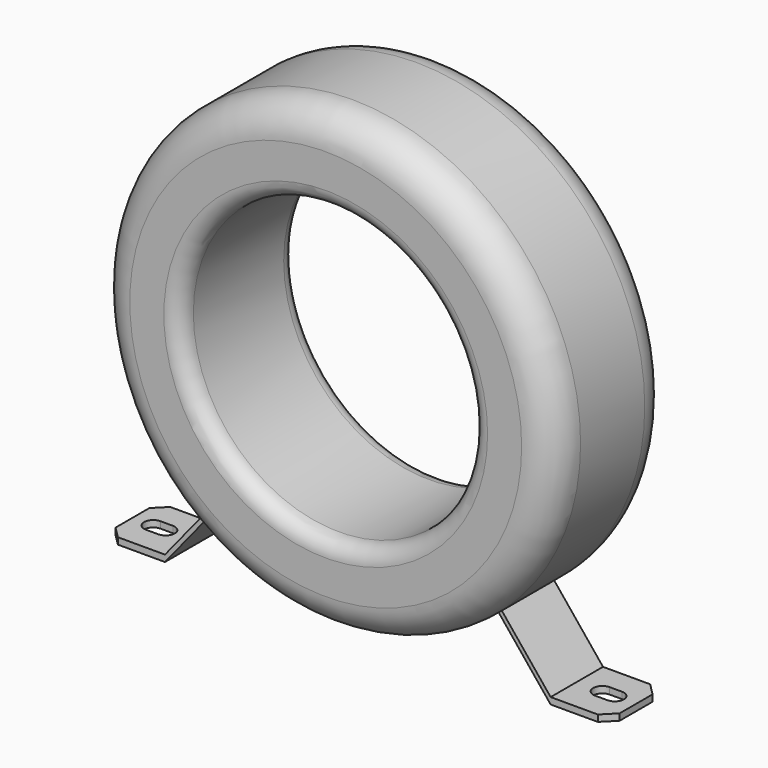
from build123d import *

# Parameters (mm, degrees)
F0_R     = 69.85
F0_R_2   = 44.45
F1_DEPTH = 22.25
F2_R     = 10
F3_R     = 5
F7_DEPTH = 2
F9_DEPTH = 20


with BuildPart() as f1:
    # F0 (on Front) → F1 (new body, symmetric)
    with BuildSketch(Plane.XZ):
        with Locations((0, 69.85)):
            Circle(F0_R)
        with Locations((0, 69.85)):
            Circle(F0_R_2, mode=Mode.SUBTRACT)
    extrude(amount=F1_DEPTH, both=True)

    # F2
    f2_edges = [f1.edges().sort_by_distance(p)[0] for p in [
        (-69.85, -22.25, 69.85),
        (-69.85, 22.25, 69.85),
    ]]
    fillet(f2_edges, radius=F2_R)

    # F3
    f3_edges = [f1.edges().sort_by_distance(p)[0] for p in [
        (-44.45, 22.25, 69.85),
        (-44.45, -22.25, 69.85),
    ]]
    fillet(f3_edges, radius=F3_R)



with BuildPart() as f7:
    # F5 (on face) → F7 (new body)
    with BuildSketch(Plane(origin=(0, 0, -4.8), x_dir=(1, 0, 0), z_dir=(0, 0, -1))):
        with BuildLine():
            Line((58.9, 10), (58.9, -10))
            Line((58.9, -10), (67.5496086478, -10))
            Line((67.5496086478, -10), (67.5496086478, -2.8))
            Line((67.5496086478, -2.8), (66.7, -2.8))
            ThreePointArc((66.7, -2.8), (63.9, 0), (66.7, 2.8))
            Line((66.7, 2.8), (67.5496086478, 2.8))
            Line((67.5496086478, 2.8), (67.5496086478, 10))
            Line((67.5496086478, 10), (58.9, 10))
        make_face()
        with BuildLine():
            Line((67.5496086478, -2.8), (67.5496086478, -10))
            Line((67.5496086478, -10), (73.3, -10))
            Line((73.3, -10), (77, -6.3))
            Line((77, -6.3), (77, 6.3))
            Line((77, 6.3), (73.3, 10))
            Line((73.3, 10), (67.5496086478, 10))
            Line((67.5496086478, 10), (67.5496086478, 2.8))
            Line((67.5496086478, 2.8), (70.5, 2.8))
            ThreePointArc((70.5, 2.8), (72.4798989873, 1.9798989873), (73.3, 0))
            ThreePointArc((73.3, 0), (72.4798989873, -1.9798989873), (70.5, -2.8))
            Line((70.5, -2.8), (67.5496086478, -2.8))
        make_face()
    extrude(amount=-F7_DEPTH)


with BuildPart() as f7b:
    # F5 (on face) → F7, piece 2 (new body)
    with BuildSketch(Plane(origin=(0, 0, -4.8), x_dir=(1, 0, 0), z_dir=(0, 0, -1))):
        Polygon((-76.8326967955, 6.4673032045), (-76.8326967955, -6.4673032045), (-73.3, -10), (-58.9, -10), (-58.9, 10), (-73.3, 10), align=None)
        with BuildLine():
            ThreePointArc((-70.5, -2.8), (-73.3, 0), (-70.5, 2.8))
            Line((-70.5, 2.8), (-66.7, 2.8))
            ThreePointArc((-66.7, 2.8), (-64.7201010127, 1.9798989873), (-63.9, 0))
            ThreePointArc((-63.9, 0), (-64.7201010127, -1.9798989873), (-66.7, -2.8))
            Line((-66.7, -2.8), (-70.5, -2.8))
        make_face(mode=Mode.SUBTRACT)
    extrude(amount=-F7_DEPTH)


with BuildPart() as f1_1:
    add(f1.part)

    add(f7.part)  # F9 merges F7

    add(f7b.part)  # F9 merges F7b
    # F8 (on face) → F9 (join, through all)
    with BuildSketch(Plane(origin=(0, 10, 0), x_dir=(-1, 0, 0), z_dir=(0, 1, 0))):
        with BuildLine():
            Line((58.9, -2.8), (43.9892310261, 15.5916360942))
            ThreePointArc((43.9892310261, 15.5916360942), (43.4982300473, 15.1972188928), (43.0036928197, 14.8072447649))
            Line((43.0036928197, 14.8072447649), (58.9, -4.8))
            Line((58.9, -4.8), (58.9, -2.8))
        make_face()
        with BuildLine():
            ThreePointArc((-43.0036928197, 14.8072447649), (-43.4982300473, 15.1972188928), (-43.9892310261, 15.5916360942))
            Line((-43.9892310261, 15.5916360942), (-58.9, -2.8))
            Line((-58.9, -2.8), (-58.9, -4.8))
            Line((-58.9, -4.8), (-43.0036928197, 14.8072447649))
        make_face()
    extrude(amount=-F9_DEPTH)


solid = f1_1.part
